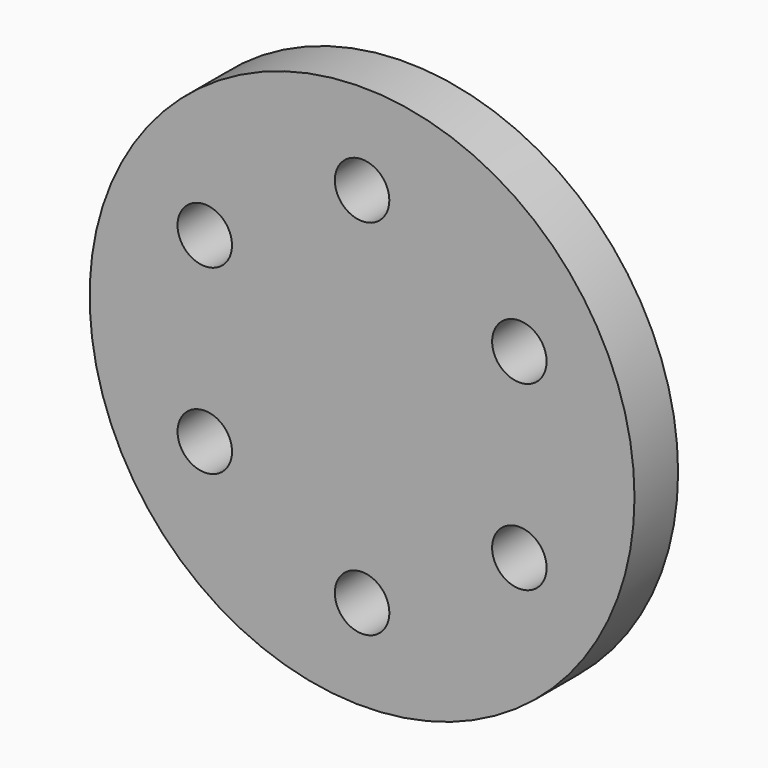
from build123d import *

# Parameters (mm, degrees)
F2_R            = 60
F3_DEPTH        = 12
F4_R            = 6
F5_DEPTH        = 12.001
F5_COPIES_COUNT = 6


# Not quite as in the source:
# - a pattern or mirror of a feature is missing from the dataset's text; its kind, count and spacing are read off the source's solid


with BuildPart() as f3:
    # F2 (on Front) → F3 (new body)
    with BuildSketch(Plane.XZ):
        Circle(F2_R)
    extrude(amount=F3_DEPTH)

    # F4 (on face) → F5 (cut, through all)
    with BuildSketch(Plane.XZ.offset(12)):
        with Locations((0, 40)):
            Circle(F4_R)
    f5 = extrude(amount=-F5_DEPTH, mode=Mode.SUBTRACT)

    # F5_copies: F5 ×6 about axis
    f5_copies_axis = Axis((0, 0, 0), (0, 1, 0))
    for i in range(1, F5_COPIES_COUNT):
        add(f5.rotate(f5_copies_axis, i * 360 / F5_COPIES_COUNT), mode=Mode.SUBTRACT)


solid = f3.part
